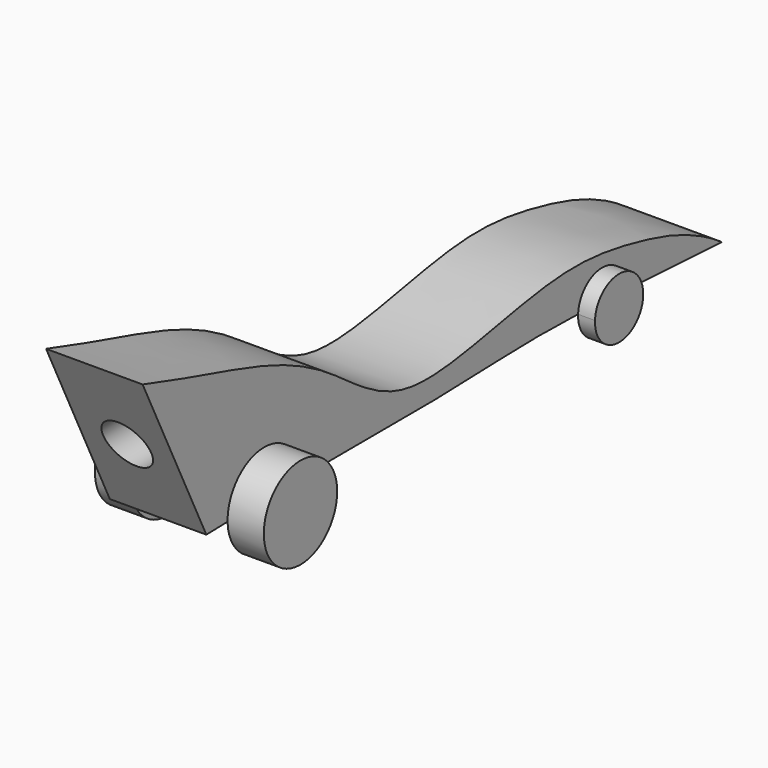
from build123d import *

# Parameters (mm, degrees)
F0_W      = 40
F0_H      = 300
F1_DEPTH  = 70
F3_DEPTH  = 40
F5_R      = 10
F6_DEPTH  = 53
F8_DEPTH  = 15
F10_DEPTH = 7


# Not quite as in the source:
# - the dataset's text gives a spline's control points without its knots; the knots are read off the source's solid
# - a feature names something its author has since deleted; it is built from what else it names


with BuildPart() as f1:
    # F0 (on Top) → F1 (new body)
    with BuildSketch(Plane.XY):
        Rectangle(F0_W, F0_H)
    extrude(amount=F1_DEPTH)

    # F2 (on face) → F3 (cut, through all)
    with BuildSketch(Plane.YZ.offset(20)):
        with BuildLine():
            Line((-150, 70), (-150, 0))
            add(Edge.make_bspline(
                [(-150, 0), (-139.0869436335, 0.8064618806), (-128.0231806764, 1.3810490807), (-116.9979503298, 1.7893701674)],
                knots=[0, 0, 0, 0, 0.083941636, 0.083941636, 0.083941636, 0.083941636], degree=3))
            Line((-116.9979503297, 1.7893701674), (-150, 70))
        make_face()
        with BuildLine():
            add(Edge.make_bspline(
                [(-150, 0), (-139.0869436335, 0.8064618806), (-128.0231806764, 1.3810490807), (-116.9979503298, 1.7893701674)],
                knots=[0, 0, 0, 0, 0.083941636, 0.083941636, 0.083941636, 0.083941636], degree=3))
            Line((-150, 0), (-116.1322072148, 0))
            Line((-116.1322072148, 0), (-116.9979503297, 1.7893701674))
        make_face()
        with BuildLine():
            Line((-116.9979503297, 1.7893701674), (-116.1322072148, 0))
            Line((-116.1322072148, 0), (150, 0))
            add(Edge.make_bspline(
                [(-116.9979503298, 1.7893701674), (-73.535565473, 3.3990062161), (4.3286680117, 1.6294165476), (61.6798983089, 6.1511100106), (120.6085361064, 1.208503553), (150, 0)],
                knots=[0.083941636, 0.083941636, 0.083941636, 0.083941636, 0.4148466214, 0.6850500549, 1, 1, 1, 1], degree=3))
        make_face()
        with BuildLine():
            Line((150, 70), (-150, 70))
            add(Edge.make_bspline(
                [(-150, 70), (-123.3503809229, 61.4840529715), (-87.6665405729, 53.2651069293), (-56.1973435382, 37.889866177), (-36.3698757715, 22.0048508877), (-12.0193448964, 9.5188468093), (25.5187784987, 14.8423564247), (69.6542827792, 24.3904520623), (107.3550399643, 18.3845533053), (134.9732802144, 10.4160223506), (150, 0)],
                knots=[0, 0, 0, 0, 0.1649237898, 0.2797560666, 0.379746261, 0.481587774, 0.6042732798, 0.7396572856, 0.8621328275, 1, 1, 1, 1], degree=3))
            Line((150, 0), (150, 70))
        make_face()
    extrude(amount=-F3_DEPTH, mode=Mode.SUBTRACT)

    # F5 (on face) → F6 (cut)
    with BuildSketch(Plane(origin=(0, -150, 0), x_dir=(-1, 0, 0), z_dir=(0, 1, 0))):
        with Locations((0, 34.789370167)):
            Circle(F5_R)
    extrude(amount=F6_DEPTH, mode=Mode.SUBTRACT)


with BuildPart() as f8:
    # F7 (on face) → F8 (new body)
    with BuildSketch(Plane.YZ.offset(20)):
        with BuildLine():
            ThreePointArc((-105.9937841102, 2.144665543), (-86.7990053561, -16.4564247346), (-67.9979503316, 2.5425336815))
            ThreePointArc((-67.9979503316, 2.5425336815), (-67.9981753753, 2.6350086021), (-67.9988505012, 2.7274813321))
            add(Edge.make_bspline(
                [(-105.9937841102, 2.144665543), (-93.0858237037, 2.5030066046), (-80.3183205464, 2.6617333769), (-67.9988505012, 2.7274813321)],
                knots=[0.1119190947, 0.1119190947, 0.1119190947, 0.1119190947, 0.210613184, 0.210613184, 0.210613184, 0.210613184], degree=3))
        make_face()
        with BuildLine():
            add(Edge.make_bspline(
                [(-105.9937841102, 2.144665543), (-93.0858237037, 2.5030066046), (-80.3183205464, 2.6617333769), (-67.9988505012, 2.7274813321)],
                knots=[0.1119190947, 0.1119190947, 0.1119190947, 0.1119190947, 0.210613184, 0.210613184, 0.210613184, 0.210613184], degree=3))
            ThreePointArc((-67.9988505012, 2.7274813321), (-87.2893628018, 21.5402987809), (-105.9937841102, 2.144665543))
        make_face()
    extrude(amount=F8_DEPTH)


with BuildPart() as f9_1:
    # F9: instance of F8
    add(f8.part.mirror(Plane.YZ))


with BuildPart() as f10:
    # F7 (on face) → F10 (new body)
    with BuildSketch(Plane.YZ.offset(20)):
        with BuildLine():
            add(Edge.make_bspline(
                [(75.5121166282, 3.9397092229), (83.4654060895, 3.6473177828), (91.8633506418, 3.2070662184), (100.4817319024, 2.7139141529)],
                knots=[0.7327089274, 0.7327089274, 0.7327089274, 0.7327089274, 0.8254400468, 0.8254400468, 0.8254400468, 0.8254400468], degree=3))
            ThreePointArc((75.5121166282, 3.9397092229), (87.3870947475, -9.0955000145), (100.4817319024, 2.7139141529))
        make_face()
        with BuildLine():
            ThreePointArc((100.5, 3.3894648293), (88.2751888921, 15.8864353051), (75.5121166282, 3.9397092229))
            add(Edge.make_bspline(
                [(75.5121166282, 3.9397092229), (83.4654060895, 3.6473177828), (91.8633506418, 3.2070662184), (100.4817319024, 2.7139141529)],
                knots=[0.7327089274, 0.7327089274, 0.7327089274, 0.7327089274, 0.8254400468, 0.8254400468, 0.8254400468, 0.8254400468], degree=3))
            ThreePointArc((100.4817319024, 2.7139141529), (100.495432141, 3.0515660131), (100.5, 3.3894648293))
        make_face()
    extrude(amount=F10_DEPTH)


with BuildPart() as f11_1:
    # F11: instance of F10
    add(f10.part.mirror(Plane.YZ))


solid = Compound([f1.part, f8.part, f9_1.part, f10.part, f11_1.part])
